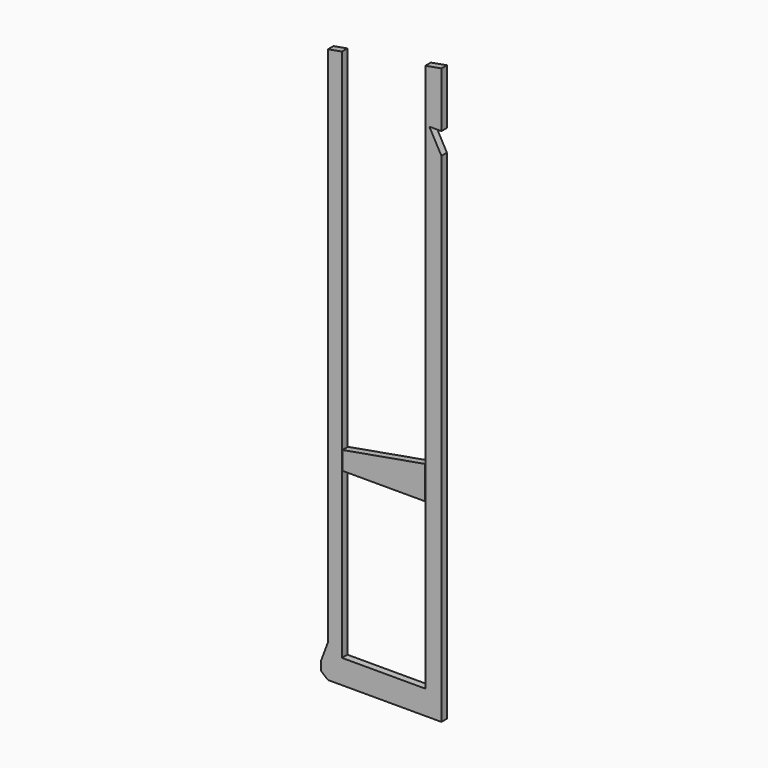
from build123d import *

# Parameters (mm, degrees)
F1_DEPTH = 3
F2_DEPTH = 3


# Not quite as in the source:
# - a feature names something its author has since deleted; it is built from what else it names


with BuildPart() as f1:
    # F0 (on Front) → F1 (new body)
    with BuildSketch(Plane.XZ):
        Polygon((-43.1878868615, -160.5870006293), (-43.1878868615, -168.5870006293), (-7.25, -168.5870006293), (-7.25, -154.250181546), align=None)
    extrude(amount=F1_DEPTH)


with BuildPart() as f2:
    # F0 (on Front) → F2 (new body)
    with BuildSketch(Plane.XZ):
        Polygon((-49.5, -251), (0, -251), (0, -33.574), (-5.25, -24.074), (0, -24.074), (0, 0), (-7, -1.234288865), (-7, -240.5024516791), (-43.4378868615, -240.5024516791), (-43.4378868615, -7.6592714386), (-49.5, -8.7281855451), (-49.5, -236.5), (-52.5, -244.5), (-52.5, -248.5), align=None)
    extrude(amount=F2_DEPTH)


solid = Compound([f1.part, f2.part])
